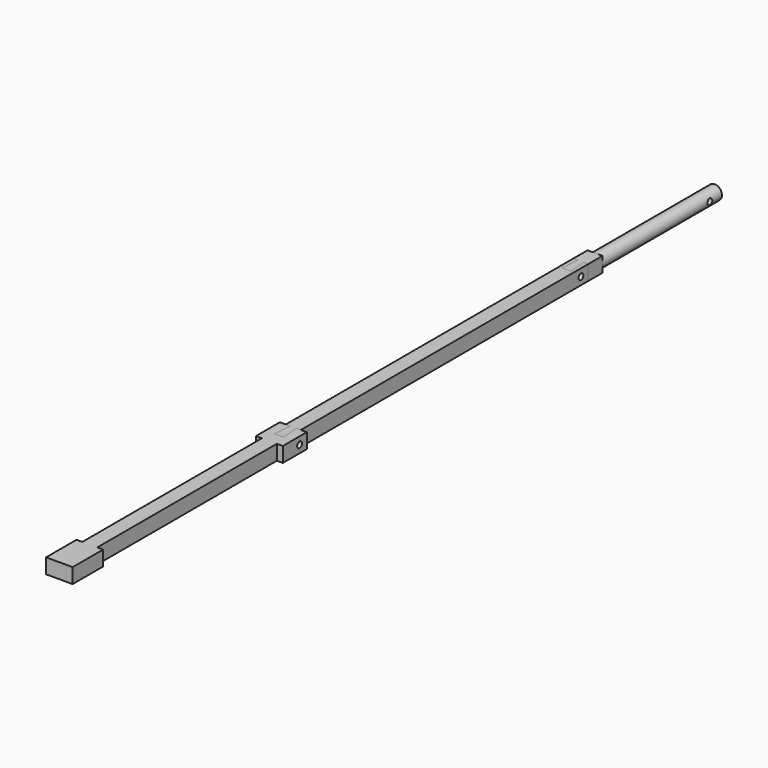
from build123d import *

# Parameters (mm, degrees)
F0_W           = 8.8713987993
F0_H           = 12.7076974937
F1_DEPTH       = 5
F2_W           = 5
F2_H           = 5
F3_DEPTH       = 85
F4_W           = 2
F4_H           = 10
F5_DEPTH       = 5
F6_DEPTH       = 5
F8_DEPTH       = 5
F9_R           = 1
F10_DEPTH      = 10
F11_R          = 1
F12_DEPTH      = 8
F12_DEPTH_BACK = 3
F13_DEPTH      = 5
F14_DEPTH      = 5
F15_R          = 2.4
F16_DEPTH      = 50
F17_R          = 1
F18_DEPTH      = 5
F19_DEPTH      = 5
F20_R          = 1
F21_DEPTH      = 5


# Not quite as in the source:
# - a feature names something its author has since deleted; it is built from what else it names


with BuildPart() as f1:
    # F0 (on Top) → F1 (new body)
    with BuildSketch(Plane.XY):
        with Locations((-2.0555156266, 32.6728799325)):
            Rectangle(F0_W, F0_H)
    extrude(amount=F1_DEPTH)

    # F2 (on face) → F3 (join)
    with BuildSketch(Plane(origin=(0, 39.0267286794, 0), x_dir=(-1, 0, 0), z_dir=(0, 1, 0))):
        with Locations((2.0555156266, 2.5)):
            Rectangle(F2_W, F2_H)
    extrude(amount=F3_DEPTH)

    # F4 (on face) → F5 (join)
    with BuildSketch(Plane.XY.offset(5)):
        with Locations((-5.5555156266, 119.0267286794)):
            Rectangle(F4_W, F4_H)
        with Locations((1.4444843734, 119.0267286794)):
            Rectangle(F4_W, F4_H)
    extrude(amount=-F5_DEPTH)

    # F4 (on face) → F6 (cut)
    with BuildSketch(Plane.XY.offset(5)):
        Polygon((-1.0555156266, 124.0267286794), (-3.0555156266, 124.0267286794), (-3.5555156266, 118.0267286794), (-0.5555156266, 118.0267286794), align=None)
    extrude(amount=-F6_DEPTH, mode=Mode.SUBTRACT)


with BuildPart() as f8:
    # F7 (on face) → F8 (new body)
    with BuildSketch(Plane.XY.offset(5)):
        Polygon((-1.0555156266, 124.0267286794), (0.4444843734, 124.0267286794), (0.4444843734, 244.0267286794), (-1.0555156266, 244.0267286794), (-0.5555156266, 238.0267286794), (-3.5555156266, 238.0267286794), (-3.0555156266, 244.0267286794), (-4.5555156266, 244.0267286794), (-4.5555156266, 124.0267286794), (-3.0555156266, 124.0267286794), (-3.5555156266, 118.0267286794), (-0.5555156266, 118.0267286794), align=None)
    extrude(amount=-F8_DEPTH)


with BuildPart() as f10_tool:
    # F9 (on face) → F10 (new body)
    with BuildSketch(Plane.YZ.offset(2.4444843734)):
        with Locations((121.0267286794, 2.5)):
            Circle(F9_R)
    extrude(amount=-F10_DEPTH)


with BuildPart() as f1_1:
    add(f1.part)

    # F10: cut by f10_tool
    add(f10_tool.part, mode=Mode.SUBTRACT)

    # F11 (on face) → F12 (cut, two sides)
    with BuildSketch(Plane.YZ.offset(0.4444843734)) as f12_sk:
        with Locations((121.0267286794, 2.5)):
            Circle(F11_R)
    extrude(amount=-F12_DEPTH, mode=Mode.SUBTRACT)
    extrude(f12_sk.sketch, amount=F12_DEPTH_BACK, mode=Mode.SUBTRACT)

    # F7 (on face) → F13 (cut)
    with BuildSketch(Plane.XY.offset(5)):
        Polygon((-1.0555156266, 244.0267286794), (0.4444843734, 244.0267286794), (0.4444843734, 250.0267286794), (-4.5555156266, 250.0267286794), (-4.5555156266, 244.0267286794), (-3.0555156266, 244.0267286794), (-3.5555156266, 238.0267286794), (-0.5555156266, 238.0267286794), align=None)
    extrude(amount=-F13_DEPTH, mode=Mode.SUBTRACT)

    # F17 (on face) → F19 (cut)
    with BuildSketch(Plane.YZ.offset(0.4444843734)):
        with Locations((241.0267286794, 2.5)):
            Circle(F17_R)
    extrude(amount=-F19_DEPTH, mode=Mode.SUBTRACT)


with BuildPart() as f8_1:
    add(f8.part)

    # F10: cut by f10_tool
    add(f10_tool.part, mode=Mode.SUBTRACT)


with BuildPart() as f14:
    # F7 (on face) → F14 (new body)
    with BuildSketch(Plane.XY.offset(5)):
        Polygon((-1.0555156266, 244.0267286794), (0.4444843734, 244.0267286794), (0.4444843734, 250.0267286794), (-4.5555156266, 250.0267286794), (-4.5555156266, 244.0267286794), (-3.0555156266, 244.0267286794), (-3.5555156266, 238.0267286794), (-0.5555156266, 238.0267286794), align=None)
    extrude(amount=-F14_DEPTH)

    # F15 (on face) → F16 (join)
    with BuildSketch(Plane(origin=(0, 250.0267286794, 0), x_dir=(-1, 0, 0), z_dir=(0, 1, 0))):
        with Locations((2.0555156266, 2.5)):
            Circle(F15_R)
    extrude(amount=F16_DEPTH)


with BuildPart() as f18_tool:
    # F17 (on face) → F18 (new body)
    with BuildSketch(Plane.YZ.offset(0.4444843734)):
        with Locations((241.0267286794, 2.5)):
            Circle(F17_R)
    extrude(amount=-F18_DEPTH)


with BuildPart() as f8_2:
    add(f8_1.part)

    # F18: cut by f18_tool
    add(f18_tool.part, mode=Mode.SUBTRACT)


with BuildPart() as f14_1:
    add(f14.part)

    # F18: cut by f18_tool
    add(f18_tool.part, mode=Mode.SUBTRACT)

    # F20 (on face) → F21 (cut)
    with BuildSketch(Plane(origin=(-4.5555156266, 0, 0), x_dir=(0, -1, 0), z_dir=(-1, 0, 0))):
        with Locations((-295.0267286794, 2.5)):
            Circle(F20_R)
    extrude(amount=-F21_DEPTH, mode=Mode.SUBTRACT)


solid = Compound([f1_1.part, f8_2.part, f14_1.part])
